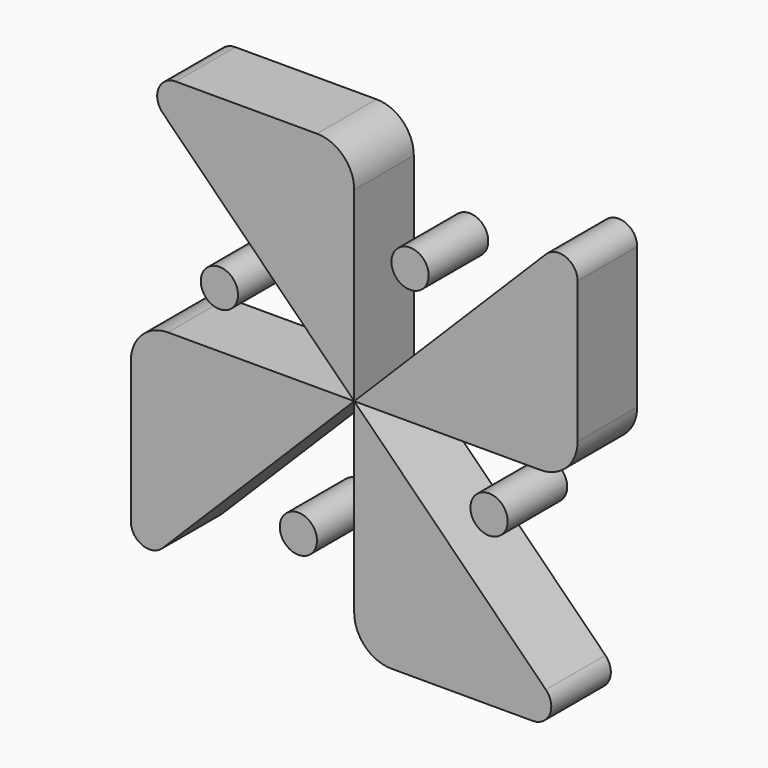
from build123d import *

# Parameters (mm, degrees)
F1_DEPTH = 25.4
F0_R     = 6.35


# Not quite as in the source:
# - the program builds the solid bodies; features that only make, move or delete a surface that nothing else refers to are left out


with BuildPart() as f1:
    # F0 (on Front) → F1 (new body)
    with BuildSketch(Plane.XZ):
        with BuildLine():
            Line((65.3598719395, 65.3598719395), (0, 0))
            Line((0, 0), (63.5, 0))
            ThreePointArc((63.5, 0), (72.4802561211, 3.7197438789), (76.2, 12.7))
            Line((76.2, 12.7), (76.2, 60.8697438789))
            ThreePointArc((76.2, 60.8697438789), (72.2800397955, 66.7363789104), (65.3598719395, 65.3598719395))
        make_face()
    extrude(amount=F1_DEPTH)


with BuildPart() as f1b:
    # F0 (on Front) → F1, piece 2 (new body)
    with BuildSketch(Plane.XZ):
        with BuildLine():
            Line((-65.3598719395, 65.3598719395), (0, 0))
            Line((0, 0), (0, 63.5))
            ThreePointArc((0, 63.5), (-3.7197438789, 72.4802561211), (-12.7, 76.2))
            Line((-12.7, 76.2), (-60.8697438789, 76.2))
            ThreePointArc((-60.8697438789, 76.2), (-66.7363789104, 72.2800397955), (-65.3598719395, 65.3598719395))
        make_face()
    extrude(amount=F1_DEPTH)


with BuildPart() as f1c:
    # F0 (on Front) → F1, piece 3 (new body)
    with BuildSketch(Plane.XZ):
        with BuildLine():
            Line((-65.3598719395, -65.3598719395), (0, 0))
            Line((0, 0), (-63.5, 0))
            ThreePointArc((-63.5, 0), (-72.4802561211, -3.7197438789), (-76.2, -12.7))
            Line((-76.2, -12.7), (-76.2, -60.8697438789))
            ThreePointArc((-76.2, -60.8697438789), (-72.2800397955, -66.7363789104), (-65.3598719395, -65.3598719395))
        make_face()
    extrude(amount=F1_DEPTH)


with BuildPart() as f1d:
    # F0 (on Front) → F1, piece 4 (new body)
    with BuildSketch(Plane.XZ):
        with BuildLine():
            Line((65.3598719395, -65.3598719395), (0, 0))
            Line((0, 0), (0, -63.5))
            ThreePointArc((0, -63.5), (3.7197438789, -72.4802561211), (12.7, -76.2))
            Line((12.7, -76.2), (60.8697438789, -76.2))
            ThreePointArc((60.8697438789, -76.2), (66.7363789104, -72.2800397955), (65.3598719395, -65.3598719395))
        make_face()
    extrude(amount=F1_DEPTH)


with BuildPart() as f1e:
    # F0 (on Front) → F1, piece 5 (new body)
    with BuildSketch(Plane.XZ):
        with Locations((-45.9907683632, 19.05)):
            Circle(F0_R)
    extrude(amount=F1_DEPTH)


with BuildPart() as f1f:
    # F0 (on Front) → F1, piece 6 (new body)
    with BuildSketch(Plane.XZ):
        with Locations((19.05, 45.9907683632)):
            Circle(F0_R)
    extrude(amount=F1_DEPTH)


with BuildPart() as f1g:
    # F0 (on Front) → F1, piece 7 (new body)
    with BuildSketch(Plane.XZ):
        with Locations((45.9907683632, -19.05)):
            Circle(F0_R)
    extrude(amount=F1_DEPTH)


with BuildPart() as f1h:
    # F0 (on Front) → F1, piece 8 (new body)
    with BuildSketch(Plane.XZ):
        with Locations((-19.05, -45.9907683632)):
            Circle(F0_R)
    extrude(amount=F1_DEPTH)


solid = Compound([f1.part, f1b.part, f1c.part, f1d.part, f1e.part, f1f.part, f1g.part, f1h.part])
